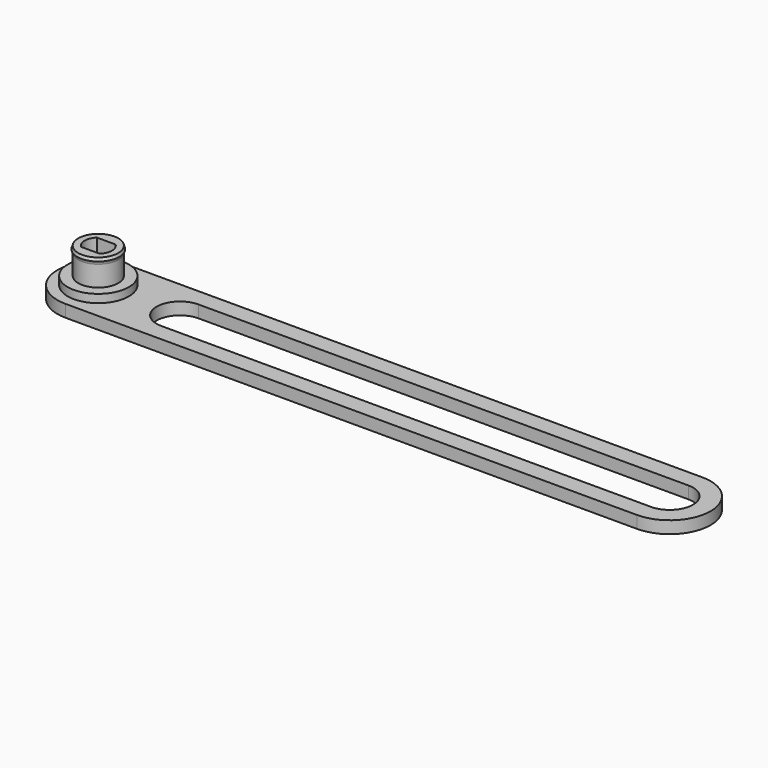
from build123d import *

# Parameters (mm, degrees)
F1_R     = 7.5
F2_DEPTH = 3
F1_R_2   = 4.9
F3_DEPTH = 5
F4_DEPTH = 11.5


# Not quite as in the source:
# - a feature names something its author has since deleted; it is built from what else it names


with BuildPart() as f2:
    # F1 (on Top) → F2 (new body)
    with BuildSketch(Plane.XY):
        with BuildLine():
            Line((120, 10), (0, 10))
            ThreePointArc((0, 10), (-10, 0), (0, -10))
            Line((0, -10), (120, -10))
            Line((120, -10), (140, -10))
            ThreePointArc((140, -10), (150, 0), (140, 10))
            Line((140, 10), (120, 10))
        make_face()
        Circle(F1_R, mode=Mode.SUBTRACT)
        with BuildLine():
            ThreePointArc((20, -5.7), (14.3, 0), (20, 5.7))
            Line((20, 5.7), (120, 5.7))
            Line((120, 5.7), (140, 5.7))
            ThreePointArc((140, 5.7), (145.7, 0), (140, -5.7))
            Line((140, -5.7), (120, -5.7))
            Line((120, -5.7), (20, -5.7))
        make_face(mode=Mode.SUBTRACT)
    extrude(amount=F2_DEPTH)

    # F1 (on Top) → F3 (join)
    with BuildSketch(Plane.XY):
        Circle(F1_R)
        Circle(F1_R_2, mode=Mode.SUBTRACT)
    extrude(amount=F3_DEPTH)

    # F1 (on Top) → F4 (join)
    with BuildSketch(Plane.XY):
        Circle(F1_R_2)
        with BuildLine():
            Line((2.2847319318, -2.45), (0, -2.45))
            Line((0, -2.45), (-2.2847319318, -2.45))
            ThreePointArc((-2.2847319318, -2.45), (-3.35, 0), (-2.2847319318, 2.45))
            Line((-2.2847319318, 2.45), (0, 2.45))
            Line((0, 2.45), (2.2847319318, 2.45))
            ThreePointArc((2.2847319318, 2.45), (3.35, 0), (2.2847319318, -2.45))
        make_face(mode=Mode.SUBTRACT)
    extrude(amount=F4_DEPTH)

    # F6 (on plane+point) → F7 (revolve)
    with BuildSketch(Plane.XZ):
        Polygon((5.15, 10.75), (4.9, 11.5), (4.9, 10), align=None)
    revolve(axis=Axis((0, 0, 5.75), (0, 0, 1)))


solid = f2.part
